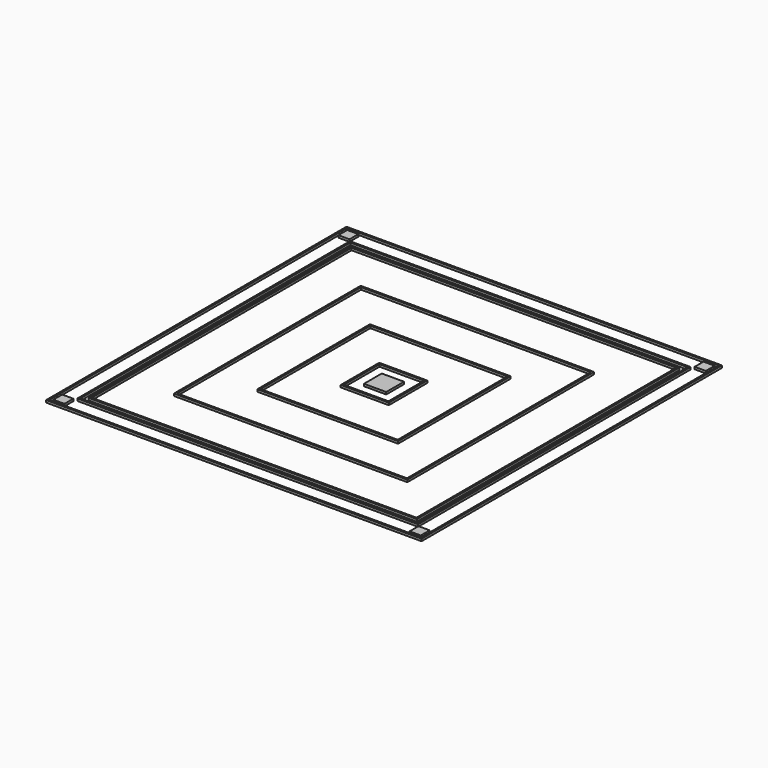
from build123d import *

# Parameters (mm, degrees)
F0_W     = 168.6
F0_H     = 168.6
F0_W_2   = 167
F0_H_2   = 167
F1_DEPTH = 1
F0_W_3   = 5
F0_H_3   = 5
F0_W_4   = 153
F0_H_4   = 153
F0_W_5   = 151.4
F0_H_5   = 151.4
F0_W_6   = 147.4
F0_H_6   = 147.4
F0_W_7   = 145.8
F0_H_7   = 145.8
F0_W_8   = 104.8
F0_H_8   = 104.8
F0_W_9   = 103.2
F0_H_9   = 103.2
F0_W_10  = 63.2
F0_H_10  = 63.2
F0_W_11  = 61.6
F0_H_11  = 61.6
F0_W_12  = 21.6
F0_H_12  = 21.6
F0_W_13  = 20
F0_H_13  = 20
F0_W_14  = 10
F0_H_14  = 10


# Not quite as in the source:
# - a feature names something its author has since deleted; it is built from what else it names


with BuildPart() as f1:
    # F0 (on Top) → F1 (new body)
    with BuildSketch(Plane.XY):
        Rectangle(F0_W, F0_H)
        Rectangle(F0_W_2, F0_H_2, mode=Mode.SUBTRACT)
    extrude(amount=F1_DEPTH)


with BuildPart() as f1b:
    # F0 (on Top) → F1, piece 2 (new body)
    with BuildSketch(Plane.XY):
        with Locations((-80, 80)):
            Rectangle(F0_W_3, F0_H_3)
    extrude(amount=F1_DEPTH)


with BuildPart() as f1c:
    # F0 (on Top) → F1, piece 3 (new body)
    with BuildSketch(Plane.XY):
        Rectangle(F0_W_4, F0_H_4)
        Rectangle(F0_W_5, F0_H_5, mode=Mode.SUBTRACT)
    extrude(amount=F1_DEPTH)


with BuildPart() as f1d:
    # F0 (on Top) → F1, piece 4 (new body)
    with BuildSketch(Plane.XY):
        Rectangle(F0_W_6, F0_H_6)
        Rectangle(F0_W_7, F0_H_7, mode=Mode.SUBTRACT)
    extrude(amount=F1_DEPTH)


with BuildPart() as f1e:
    # F0 (on Top) → F1, piece 5 (new body)
    with BuildSketch(Plane.XY):
        Rectangle(F0_W_8, F0_H_8)
        Rectangle(F0_W_9, F0_H_9, mode=Mode.SUBTRACT)
    extrude(amount=F1_DEPTH)


with BuildPart() as f1f:
    # F0 (on Top) → F1, piece 6 (new body)
    with BuildSketch(Plane.XY):
        Rectangle(F0_W_10, F0_H_10)
        Rectangle(F0_W_11, F0_H_11, mode=Mode.SUBTRACT)
    extrude(amount=F1_DEPTH)


with BuildPart() as f1g:
    # F0 (on Top) → F1, piece 7 (new body)
    with BuildSketch(Plane.XY):
        Rectangle(F0_W_12, F0_H_12)
        Rectangle(F0_W_13, F0_H_13, mode=Mode.SUBTRACT)
    extrude(amount=F1_DEPTH)


with BuildPart() as f1h:
    # F0 (on Top) → F1, piece 8 (new body)
    with BuildSketch(Plane.XY):
        Rectangle(F0_W_14, F0_H_14)
    extrude(amount=F1_DEPTH)


with BuildPart() as f1i:
    # F0 (on Top) → F1, piece 9 (new body)
    with BuildSketch(Plane.XY):
        with Locations((80, 80)):
            Rectangle(F0_W_3, F0_H_3)
    extrude(amount=F1_DEPTH)


with BuildPart() as f1j:
    # F0 (on Top) → F1, piece 10 (new body)
    with BuildSketch(Plane.XY):
        Polygon((77.5, -77.5), (77.5, -80), (77.5, -82.5), (82.5, -82.5), (82.5, -77.5), align=None)
    extrude(amount=F1_DEPTH)


with BuildPart() as f1k:
    # F0 (on Top) → F1, piece 11 (new body)
    with BuildSketch(Plane.XY):
        Polygon((-77.5, -77.5), (-82.5, -77.5), (-82.5, -82.5), (-77.5, -82.5), (-77.5, -80), align=None)
    extrude(amount=F1_DEPTH)


solid = Compound([f1.part, f1b.part, f1c.part, f1d.part, f1e.part, f1f.part, f1g.part, f1h.part, f1i.part, f1j.part, f1k.part])
